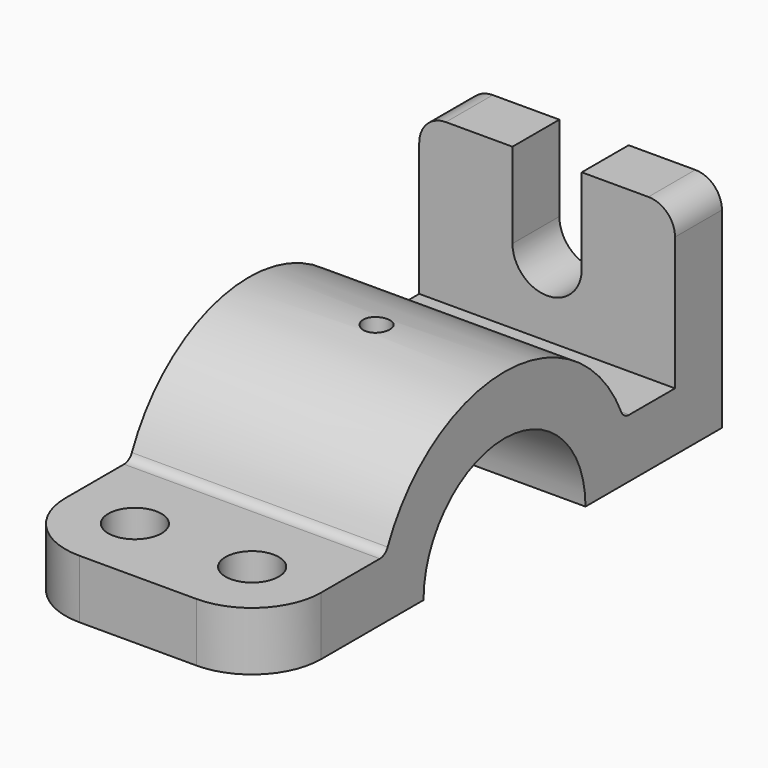
from build123d import *

# Parameters (mm, degrees)
F0_W     = 11
F0_H     = 30
F1_DEPTH = 24
F3_DEPTH = 11
F4_R     = 5
F4_R_2   = 2.5
F5_DEPTH = 41.001
F6_R     = 13
F7_R     = 5
F8_R     = 2


# Not quite as in the source:
# - ends of sketch curves that miss each other by under 0.0002 mm in the source are joined


with BuildPart() as f1:
    # F0 (on Right) → F1 (new body, symmetric)
    with BuildSketch(Plane.YZ):
        with BuildLine():
            Line((-56, 0), (-30, 0))
            ThreePointArc((-30, 0), (-29.4730143031, 5.5983415304), (-27.9105714739, 11))
            Line((-27.9105714739, 11), (-56, 11))
            Line((-56, 11), (-56, 0))
        make_face()
        with BuildLine():
            Line((-30, 0), (-19, 0))
            ThreePointArc((-19, 0), (-18.1017503893, 5.7729223833), (-15.4919333848, 11))
            Line((-15.4919333848, 11), (-27.9105714739, 11))
            ThreePointArc((-27.9105714739, 11), (-29.4730143031, 5.5983415304), (-30, 0))
        make_face()
        with BuildLine():
            ThreePointArc((-15.4919333848, 11), (0, 19), (15.4919333848, 11))
            Line((15.4919333848, 11), (27.9105714739, 11))
            ThreePointArc((27.9105714739, 11), (0, 30), (-27.9105714739, 11))
            Line((-27.9105714739, 11), (-15.4919333848, 11))
        make_face()
        with BuildLine():
            ThreePointArc((15.4919333848, 11), (18.1017503893, 5.7729223833), (19, 0))
            Line((19, 0), (30, 0))
            ThreePointArc((30, 0), (29.4730143031, 5.5983415304), (27.9105714739, 11))
            Line((27.9105714739, 11), (15.4919333848, 11))
        make_face()
        with BuildLine():
            ThreePointArc((27.9105714739, 11), (29.4730143031, 5.5983415304), (30, 0))
            Line((30, 0), (51, 0))
            Line((51, 0), (51, 11))
            Line((51, 11), (40, 11))
            Line((40, 11), (27.9105714739, 11))
        make_face()
        with Locations((45.5, 26)):
            Rectangle(F0_W, F0_H)
    extrude(amount=F1_DEPTH, both=True)

    # F2 (on face) → F3 (cut, through all)
    with BuildSketch(Plane(origin=(0, 51, 0), x_dir=(-1, 0, 0), z_dir=(0, 1, 0))):
        with BuildLine():
            Line((-6.4943742253, 25.2703764435), (-6.4943742253, 24.7296235565))
            ThreePointArc((-6.4943742253, 24.7296235565), (0.1340750741, 18.501382926), (6.4999995983, 24.9977146924))
            ThreePointArc((6.4999995983, 24.9977146924), (6.4999998996, 24.9988573462), (6.5, 25))
            ThreePointArc((6.5, 25), (0.1352174827, 31.4985934041), (-6.4943742253, 25.2703764435))
        make_face()
        with BuildLine():
            Line((-6.4943742253, 41), (-6.4943742253, 25.2703764435))
            ThreePointArc((-6.4943742253, 25.2703764435), (0.1352174827, 31.4985934041), (6.5, 25))
            Line((6.5, 25), (6.5056257747, 41))
            Line((6.5056257747, 41), (-6.4943742253, 41))
        make_face()
    extrude(amount=-F3_DEPTH, mode=Mode.SUBTRACT)

    # F4 (on Top) → F5 (cut, through all)
    with BuildSketch(Plane.XY):
        with Locations((11, -42.9459065199)):
            Circle(F4_R)
        with Locations((-11, -42.9459065199)):
            Circle(F4_R)
        Circle(F4_R_2)
    extrude(amount=F5_DEPTH, mode=Mode.SUBTRACT)

    # F6
    f6_edges = [f1.edges().sort_by_distance(p)[0] for p in [
        (-24, -56, 5.5),
        (24, -56, 5.5),
    ]]
    fillet(f6_edges, radius=F6_R)

    # F7
    f7_edges = [f1.edges().sort_by_distance(p)[0] for p in [
        (-24, 45.5, 41),
        (24, 45.5, 41),
    ]]
    fillet(f7_edges, radius=F7_R)

    # F8
    f8_edges = [f1.edges().sort_by_distance(p)[0] for p in [
        (0, -27.910571, 11),
        (0, 27.910571, 11),
    ]]
    fillet(f8_edges, radius=F8_R)


solid = f1.part
